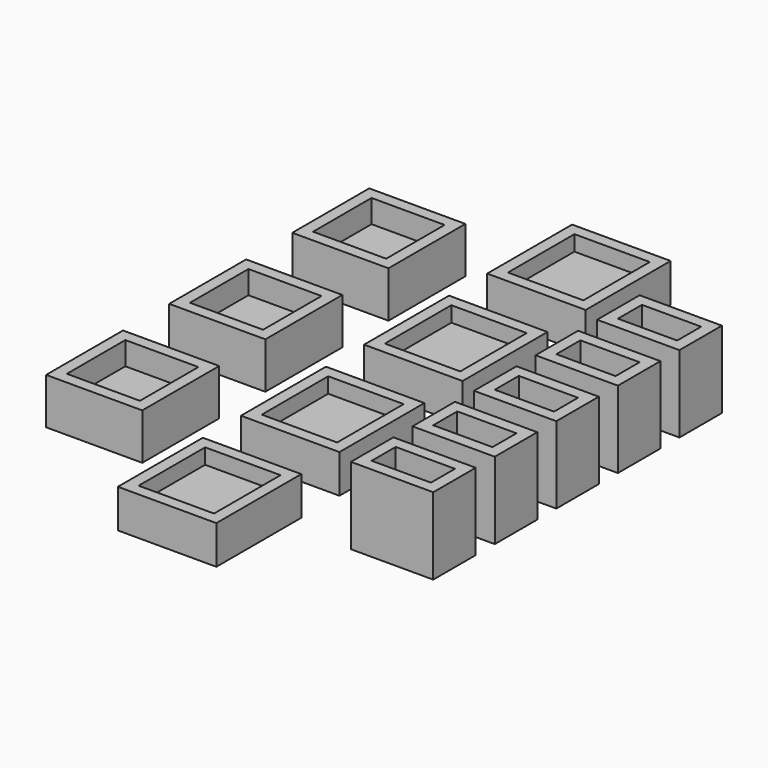
from build123d import *

# Parameters (mm, degrees)
F0_W          = 10.7
F0_H          = 6.9
F1_DEPTH      = 10
F2_W          = 7.7
F2_H          = 3.9
F3_DEPTH      = 7
F6_TEXT_SIZE  = 6.0464025915
F7_DEPTH      = 2
F10_W         = 12.5
F10_H         = 12.5
F11_DEPTH     = 6
F12_W         = 9.5
F12_H         = 9.5
F13_DEPTH     = 3
F15_TEXT_SIZE = 8.6785300583
F16_DEPTH     = 2
F18_ANGLE     = 180
F19_ANGLE     = 180
F31_W         = 12.8
F31_H         = 13.8
F32_DEPTH     = 5
F33_W         = 9.8
F33_H         = 10.8
F34_DEPTH     = 2
F37_TEXT_SIZE = 9.6995331761
F38_DEPTH     = 2


# Not quite as in the source:
# - Text() gives the source's letters only with a copy of the font that has no kerning and outlines rounded to 1/6400 em; it was checked with that copy


with BuildPart() as f1:
    # F0 (on Top) → F1 (new body)
    with BuildSketch(Plane.XY):
        Rectangle(F0_W, F0_H)
    extrude(amount=F1_DEPTH)


with BuildPart() as f3:
    # F2 (on Top) → F3 (new body)
    with BuildSketch(Plane.XY):
        Rectangle(F2_W, F2_H)
    extrude(amount=F3_DEPTH)


with BuildPart() as f1_1:
    add(f1.part)

    # F4: cut F3
    add(f3.part, mode=Mode.SUBTRACT)


with BuildPart() as f1_2:
    # F5: moved
    add(f1_1.part.moved(Location((20, 0, 0))))


with BuildPart() as f7:
    # F6 (on face) → F7 (new body)
    with BuildSketch(Plane.XY.offset(10)):
        with Locations((19.7949353606, -1.7978313845)):
            Text('A', F6_TEXT_SIZE, font='Open Sans', font_style=FontStyle.BOLD, text_align=(TextAlign.LEFT, TextAlign.BOTTOM))
    extrude(amount=-F7_DEPTH)


with BuildPart() as f7_1:
    # F8: moved
    add(f7.part.moved(Location((-2, 0, 0))))


with BuildPart() as f1_3:
    add(f1_2.part)

    # F9: cut F7
    add(f7_1.part, mode=Mode.SUBTRACT)


with BuildPart() as f11:
    # F10 (on Top) → F11 (new body)
    with BuildSketch(Plane.XY):
        Rectangle(F10_W, F10_H)
    extrude(amount=F11_DEPTH)


with BuildPart() as f13:
    # F12 (on Top) → F13 (new body)
    with BuildSketch(Plane.XY):
        Rectangle(F12_W, F12_H)
    extrude(amount=F13_DEPTH)


with BuildPart() as f11_1:
    add(f11.part)

    # F14: cut F13
    add(f13.part, mode=Mode.SUBTRACT)


with BuildPart() as f16:
    # F15 (on face) → F16 (new body)
    with BuildSketch(Plane.XY.offset(6)):
        with Locations((-2.9404903762, -3.2161611598)):
            Text('B', F15_TEXT_SIZE, font='Open Sans', font_style=FontStyle.BOLD, text_align=(TextAlign.LEFT, TextAlign.BOTTOM))
    extrude(amount=-F16_DEPTH)


with BuildPart() as f11_2:
    add(f11_1.part)

    # F17: cut F16
    add(f16.part, mode=Mode.SUBTRACT)


with BuildPart() as f1_4:
    # F18: moved
    add(f1_3.part.rotate(Axis((20, -3.45, 0), (-1, 0, 0)), F18_ANGLE))


with BuildPart() as f11_3:
    # F19: moved
    add(f11_2.part.rotate(Axis((0, -6.25, 0), (1, 0, 0)), F19_ANGLE))


with BuildPart() as f11_4:
    # F20: moved
    add(f11_3.part.moved(Location((0, 0, 6))))


with BuildPart() as f1_5:
    # F21: moved
    add(f1_4.part.moved(Location((0, 0, 10))))


with BuildPart() as f22_1:
    # F22: copy of F1
    add(f1_5.part.moved(Location((0, 10, 0))))


with BuildPart() as f23_1:
    # F23: copy of F1
    add(f1_5.part.moved(Location((0, -10, 0))))


with BuildPart() as f23_1_1:
    # F24: moved
    add(f23_1.part.moved(Location((0, 0, -10))))


with BuildPart() as f25_1:
    # F25: copy of F23_1
    add(f23_1_1.part.moved(Location((0, -10, 0))))


with BuildPart() as f22_1_1:
    # F26: moved
    add(f22_1.part.moved(Location((0, 10, 0))))


with BuildPart() as f27_1:
    # F27: copy of F22_1
    add(f22_1_1.part.moved(Location((0, -10, 0))))


with BuildPart() as f28_1:
    # F28: copy of F11
    add(f11_4.part.moved(Location((0, 20, 0))))


with BuildPart() as f29_1:
    # F29: copy of F11
    add(f11_4.part.moved(Location((0, -20, 0))))


with BuildPart() as f29_1_1:
    # F30: moved
    add(f29_1.part.moved(Location((-20, 10, 0))))


with BuildPart() as f28_1_1:
    # F30: moved
    add(f28_1.part.moved(Location((-20, 10, 0))))


with BuildPart() as f11_5:
    # F30: moved
    add(f11_4.part.moved(Location((-20, 10, 0))))


with BuildPart() as f32:
    # F31 (on Top) → F32 (new body)
    with BuildSketch(Plane.XY):
        Rectangle(F31_W, F31_H)
    extrude(amount=F32_DEPTH)


with BuildPart() as f34:
    # F33 (on face) → F34 (new body)
    with BuildSketch(Plane.XY.offset(5)):
        Rectangle(F33_W, F33_H)
    extrude(amount=-F34_DEPTH)


with BuildPart() as f32_1:
    add(f32.part)

    # F35: cut F34
    add(f34.part, mode=Mode.SUBTRACT)


with BuildPart() as f23_1_2:
    # F36: moved
    add(f23_1_1.part.moved(Location((0, 0, 10))))


with BuildPart() as f25_1_1:
    # F36: moved
    add(f25_1.part.moved(Location((0, 0, 10))))


with BuildPart() as f38:
    # F37 (on face) → F38 (new body)
    with BuildSketch(Plane(origin=(0, 0, 0), x_dir=(1, 0, 0), z_dir=(0, 0, -1))):
        with Locations((-2.9404903762, -3.5837222822)):
            Text('C', F37_TEXT_SIZE, font='Open Sans', font_style=FontStyle.BOLD, text_align=(TextAlign.LEFT, TextAlign.BOTTOM))
    extrude(amount=-F38_DEPTH)


with BuildPart() as f32_2:
    add(f32_1.part)

    # F39: cut F38
    add(f38.part, mode=Mode.SUBTRACT)


with BuildPart() as f40_1:
    # F40: copy of F32
    add(f32_2.part.moved(Location((0, -20, 0))))


with BuildPart() as f41_1:
    # F41: copy of F32
    add(f32_2.part.moved(Location((0, 40, 0))))


with BuildPart() as f41_2:
    # F41: copy of F40_1
    add(f40_1.part.moved(Location((0, 40, 0))))


with BuildPart() as f32_3:
    # F42: moved
    add(f32_2.part.moved(Location((0, -15, 0))))


with BuildPart() as f40_1_1:
    # F42: moved
    add(f40_1.part.moved(Location((0, -15, 0))))


with BuildPart() as f41_1_1:
    # F42: moved
    add(f41_1.part.moved(Location((0, -15, 0))))


with BuildPart() as f41_2_1:
    # F42: moved
    add(f41_2.part.moved(Location((0, -15, 0))))


solid = Compound([f1_5.part, f22_1_1.part, f27_1.part, f29_1_1.part, f28_1_1.part, f11_5.part, f23_1_2.part, f25_1_1.part, f32_3.part, f40_1_1.part, f41_1_1.part, f41_2_1.part])
